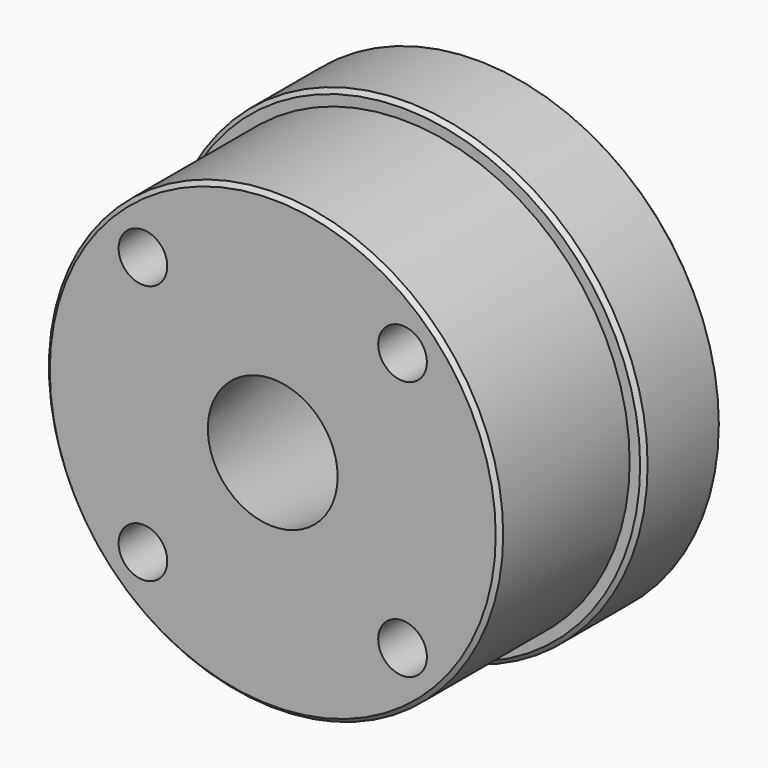
from build123d import *

# Parameters (mm, degrees)
F0_R     = 47.3075
F0_R_2   = 44.45
F1_DEPTH = 19.05
F0_R_3   = 12.7
F2_DEPTH = 50.8
F3_SIZE2 = 7.139464
F3_SIZE  = 50.79999
F4_R     = 26.9875
F4_R_2   = 12.7
F5_DEPTH = 2.921
F7_D     = 9.525
F7_DEPTH = 19.05
F7_TIP   = 2.8615986981
F8_SIZE  = 0.8128


# Not quite as in the source:
# - a fillet or chamfer is up to 0.001 mm smaller than in the source, because OpenCascade refuses the exact size


with BuildPart() as f1:
    # F0 (on Front) → F1 (new body)
    with BuildSketch(Plane.XZ):
        Circle(F0_R)
        Circle(F0_R_2, mode=Mode.SUBTRACT)
    extrude(amount=F1_DEPTH)

    # F0 (on Front) → F2 (join)
    with BuildSketch(Plane.XZ):
        Circle(F0_R_2)
        Circle(F0_R_3, mode=Mode.SUBTRACT)
    extrude(amount=F2_DEPTH)

    # F3 (size 50.8 and 7.1394744029 in the source; OpenCascade refuses exactly that, so slightly less here)
    f3_edges = [f1.edges().sort_by_distance(p)[0] for p in [
        (-12.7, 0, 0),
    ]]
    f3_side = f1.faces().sort_by_distance((-12.7, -25.4, 0))[0]
    chamfer(f3_edges, length=F3_SIZE, length2=F3_SIZE2, reference=f3_side)

    # F4 (on face) → F5 (cut)
    with BuildSketch(Plane.XZ):
        Circle(F4_R)
        Circle(F4_R_2, mode=Mode.SUBTRACT)
    extrude(amount=F5_DEPTH, mode=Mode.SUBTRACT)

    # F7
    with Locations(Plane.XZ.offset(50.8)):
        with Locations((-25.4, 25.4), (25.4, 25.4), (-25.4, -25.4), (25.4, -25.4)):
            Hole(F7_D / 2, depth=F7_DEPTH)
            with Locations((0, 0, -(F7_DEPTH + F7_TIP / 2))):  # 118° drill point
                Cone(0, F7_D / 2, F7_TIP, mode=Mode.SUBTRACT)

    # F8
    f8_edges = [f1.edges().sort_by_distance(p)[0] for p in [
        (-44.45, -50.8, 0),
        (-47.3075, -19.05, 0),
        (-47.3075, 0, 0),
    ]]
    chamfer(f8_edges, length=F8_SIZE)


solid = f1.part
